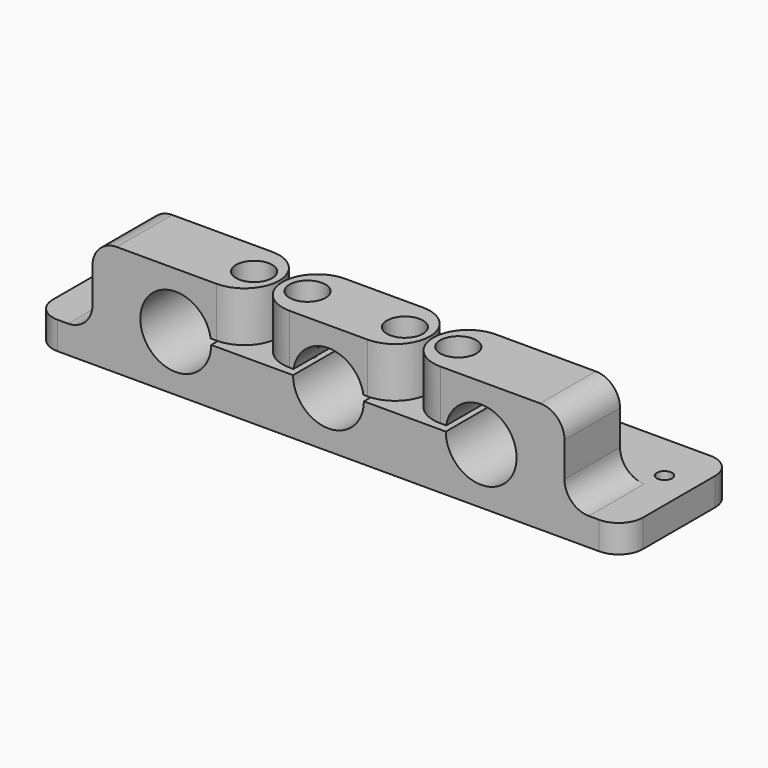
from build123d import *

# Parameters (mm, degrees)
F0_W      = 85
F0_H      = 16
F0_R      = 5.1
F1_DEPTH  = 20
F2_W      = 68
F2_H      = 10
F3_DEPTH  = 12
F4_W      = 0.4902059005
F4_H      = 7.2
F5_DEPTH  = 25
F6_R      = 3.5
F7_R      = 1.1
F8_DEPTH  = 25
F9_R      = 4.99999
F10_R     = 1.1
F11_DEPTH = 25
F12_R     = 2.6
F12_R_2   = 1.1
F13_DEPTH = 6


# Not quite as in the source:
# - a fillet or chamfer is up to 0.001 mm smaller than in the source, because OpenCascade refuses the exact size


with BuildPart() as f1:
    # F0 (on Front) → F1 (new body)
    with BuildSketch(Plane.XZ):
        Rectangle(F0_W, F0_H)
        with Locations((-22, 0)):
            Circle(F0_R, mode=Mode.SUBTRACT)
        Circle(F0_R, mode=Mode.SUBTRACT)
        with Locations((22, 0)):
            Circle(F0_R, mode=Mode.SUBTRACT)
    extrude(amount=F1_DEPTH)

    # F2 (on face) → F3 (cut)
    with BuildSketch(Plane.XY.offset(8)):
        Polygon((42.5, -20), (42.5, 0), (34, 0), (34, -10), (34, -20), align=None)
        with Locations((0, -5)):
            Rectangle(F2_W, F2_H)
        Polygon((-34, -10), (-34, 0), (-42.5, 0), (-42.5, -20), (-34, -20), align=None)
    extrude(amount=-F3_DEPTH, mode=Mode.SUBTRACT)

    # F4 (on face) → F5 (cut)
    with BuildSketch(Plane.XZ.offset(20)):
        Polygon((-11.1030349508, 0.8), (-17.6240189229, 0.8), (-17.6240189229, 0), (-3.6016391778, 0), (-3.6016391778, 0.8), (-10.6128290503, 0.8), align=None)
        with Locations((-10.8579320006, 4.4)):
            Rectangle(F4_W, F4_H)
        Polygon((4.212562261, 0.8), (4.212562261, 0), (21.7539005794, 0), (21.7539005794, 0.8), (11.1030349508, 0.8), (10.6128290503, 0.8), align=None)
        with Locations((10.8579320006, 4.4)):
            Rectangle(F4_W, F4_H)
    extrude(amount=-F5_DEPTH, mode=Mode.SUBTRACT)

    # F6
    f6_edges = [f1.edges().sort_by_distance(p)[0] for p in [
        (-34, -15, 8),
        (34, -15, 8),
        (-34, -15, -4),
        (34, -15, -4),
        (-42.5, -20, -6),
        (-42.5, 0, -6),
        (42.5, -20, -6),
        (42.5, 0, -6),
        (11, -10, -4),
        (-11, -10, -4),
    ]]
    fillet(f6_edges, radius=F6_R)

    # F7 (on face) → F8 (cut)
    with BuildSketch(Plane.XY.offset(8)):
        with Locations((-14.7030349508, -15)):
            Circle(F7_R)
        with Locations((-7.0128290503, -15)):
            Circle(F7_R)
        with Locations((7.0128290503, -15)):
            Circle(F7_R)
        with Locations((14.7030349508, -15)):
            Circle(F7_R)
    extrude(amount=-F8_DEPTH, mode=Mode.SUBTRACT)

    # F9 (radius 5 in the source; OpenCascade refuses exactly that, so slightly less here)
    f9_edges = [f1.edges().sort_by_distance(p)[0] for p in [
        (-11.103035, -20, 4.4),
        (-10.612829, -20, 4.4),
        (10.612829, -20, 4.4),
        (11.103035, -20, 4.4),
        (11.103035, -10, 4.4),
        (10.612829, -10, 4.4),
        (-10.612829, -10, 4.4),
        (-11.103035, -10, 4.4),
    ]]
    fillet(f9_edges, radius=F9_R)

    # F10 (on face) → F11 (cut)
    with BuildSketch(Plane.XY.offset(-4)):
        with Locations((38, -7)):
            Circle(F10_R)
        with Locations((-38, -7)):
            Circle(F10_R)
    extrude(amount=-F11_DEPTH, mode=Mode.SUBTRACT)

    # F12 (on face) → F13 (cut)
    with BuildSketch(Plane.XY.offset(8)):
        with Locations((-14.7030349508, -15)):
            Circle(F12_R)
        with Locations((-7.0128290503, -15)):
            Circle(F12_R)
        with Locations((-7.0128290503, -15)):
            Circle(F12_R_2, mode=Mode.SUBTRACT)
        with Locations((7.0128290503, -15)):
            Circle(F12_R)
        with Locations((7.0128290503, -15)):
            Circle(F12_R_2, mode=Mode.SUBTRACT)
        with Locations((14.7030349508, -15)):
            Circle(F12_R)
    extrude(amount=-F13_DEPTH, mode=Mode.SUBTRACT)


solid = f1.part
